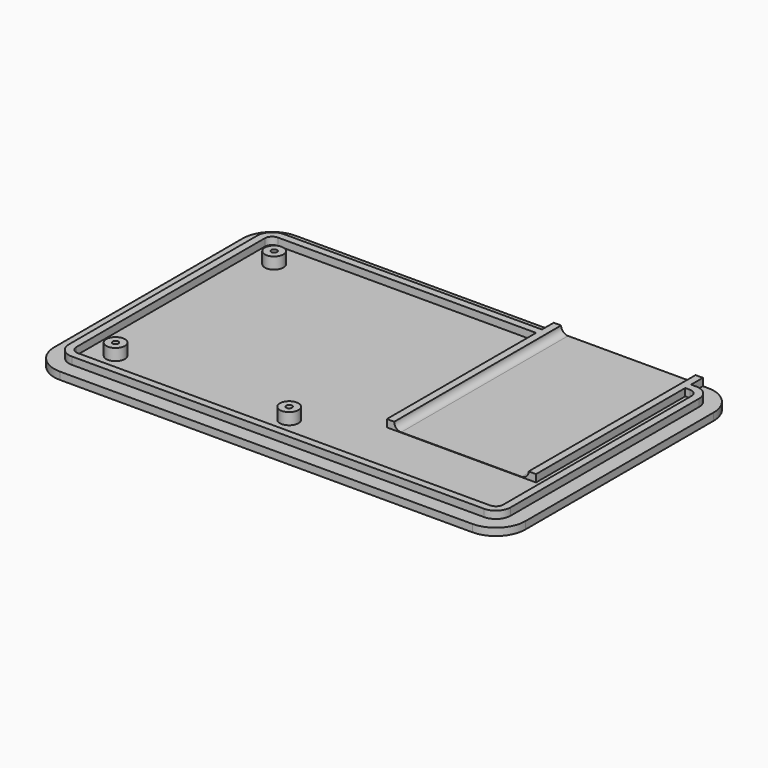
from build123d import *

# Parameters (mm, degrees)
F0_W             = 203.2
F0_H             = 127
F1_DEPTH         = 3.175
F2_R             = 12.7
F4_DEPTH         = 3.175
F5_T             = -3.175
F6_W             = 58
F6_H             = 9.525
F7_DEPTH         = 3.176
F9_DEPTH         = 90
F10_DEPTH        = 3.175
F11_DEPTH        = 3.175
F12_R            = 4
F13_DEPTH        = 5
F17_D            = 2.5
F17_DEPTH        = 5
F17_TIP          = 0.7510757738
F17_ON_F15_D     = 2.5
F17_ON_F15_DEPTH = 5
F17_ON_F15_TIP   = 0.7510757738
F17_ON_F16_D     = 2.5
F17_ON_F16_DEPTH = 5
F17_ON_F16_TIP   = 0.7510757738


# Not quite as in the source:
# - a feature names something its author has since deleted; it is built from what else it names


with BuildPart() as f1:
    # F0 (on Top) → F1 (new body)
    with BuildSketch(Plane.XY):
        Rectangle(F0_W, F0_H)
    extrude(amount=F1_DEPTH)

    # F2
    f2_edges = [f1.edges().sort_by_distance(p)[0] for p in [
        (-101.6, -63.5, 1.5875),
        (-101.6, 63.5, 1.5875),
        (101.6, -63.5, 1.5875),
        (101.6, 63.5, 1.5875),
    ]]
    fillet(f2_edges, radius=F2_R)

    # F3 (on face) → F4 (join)
    with BuildSketch(Plane.XY.offset(3.175)):
        with BuildLine():
            Line((88.9, 57.15), (-88.9, 57.15))
            ThreePointArc((-88.9, 57.15), (-93.3901280605, 55.2901280605), (-95.25, 50.8))
            Line((-95.25, 50.8), (-95.25, -50.8))
            ThreePointArc((-95.25, -50.8), (-93.3901280605, -55.2901280605), (-88.9, -57.15))
            Line((-88.9, -57.15), (88.9, -57.15))
            ThreePointArc((88.9, -57.15), (93.3901280605, -55.2901280605), (95.25, -50.8))
            Line((95.25, -50.8), (95.25, 50.8))
            ThreePointArc((95.25, 50.8), (93.3901280605, 55.2901280605), (88.9, 57.15))
        make_face()
    extrude(amount=F4_DEPTH)

    # F5
    f5_openings = [f1.faces().sort_by_distance(p)[0] for p in [
        (0, 0, 6.35),
    ]]
    offset(amount=F5_T, openings=f5_openings, kind=Kind.INTERSECTION)

    # F6 (on face) → F7 (cut, through all)
    with BuildSketch(Plane.XY.offset(3.175)):
        with Locations((54.6, 58.7375)):
            Rectangle(F6_W, F6_H)
    extrude(amount=F7_DEPTH, mode=Mode.SUBTRACT)

    # F8 (on face) → F9 (join)
    with BuildSketch(Plane(origin=(0, 63.5, 0), x_dir=(-1, 0, 0), z_dir=(0, 1, 0))):
        with BuildLine():
            Line((-83.6, 6.35), (-83.6, 3.175))
            Line((-83.6, 3.175), (-25.6, 3.175))
            Line((-25.6, 3.175), (-25.6, 6.35))
            ThreePointArc((-25.6, 6.35), (-26.4786796564, 4.2286796564), (-28.6, 3.35))
            Line((-28.6, 3.35), (-80.6, 3.35))
            ThreePointArc((-80.6, 3.35), (-82.7213203436, 4.2286796564), (-83.6, 6.35))
        make_face()
    extrude(amount=-F9_DEPTH)

    # F10 (add): faces of the model
    f10_faces = [f1.faces().sort_by_distance(p)[0] for p in [
        (25.6, 13.7375, 4.7625),
        (25.6, 60.325, 4.7625),
    ]]
    extrude(f10_faces, amount=F10_DEPTH)

    # F11 (add): faces of the model
    f11_faces = [f1.faces().sort_by_distance(p)[0] for p in [
        (83.6, 13.7375, 4.7625),
        (83.6, 60.325, 4.7625),
    ]]
    extrude(f11_faces, amount=F11_DEPTH)

    # F12 (on face) → F13 (join)
    with BuildSketch(Plane.XY.offset(3.175)):
        with Locations((-81.6051200401, -42.75)):
            Circle(F12_R)
        with Locations((-6.7051200401, -42.75)):
            Circle(F12_R)
        with Locations((-81.6051200401, 42.75)):
            Circle(F12_R)
    extrude(amount=F13_DEPTH)

    # F17
    with Locations(Plane.XY.offset(8.175)):
        with Locations((-81.6051200401, 42.75)):
            Hole(F17_D / 2, depth=F17_DEPTH)
            with Locations((0, 0, -(F17_DEPTH + F17_TIP / 2))):  # 118° drill point
                Cone(0, F17_D / 2, F17_TIP, mode=Mode.SUBTRACT)

    # F17 on F15
    with Locations(Plane.XY.offset(8.175)):
        with Locations((-81.6051200401, -42.75)):
            Hole(F17_ON_F15_D / 2, depth=F17_ON_F15_DEPTH)
            with Locations((0, 0, -(F17_ON_F15_DEPTH + F17_ON_F15_TIP / 2))):  # 118° drill point
                Cone(0, F17_ON_F15_D / 2, F17_ON_F15_TIP, mode=Mode.SUBTRACT)

    # F17 on F16
    with Locations(Plane.XY.offset(8.175)):
        with Locations((-6.7051200401, -42.75)):
            Hole(F17_ON_F16_D / 2, depth=F17_ON_F16_DEPTH)
            with Locations((0, 0, -(F17_ON_F16_DEPTH + F17_ON_F16_TIP / 2))):  # 118° drill point
                Cone(0, F17_ON_F16_D / 2, F17_ON_F16_TIP, mode=Mode.SUBTRACT)


solid = f1.part
